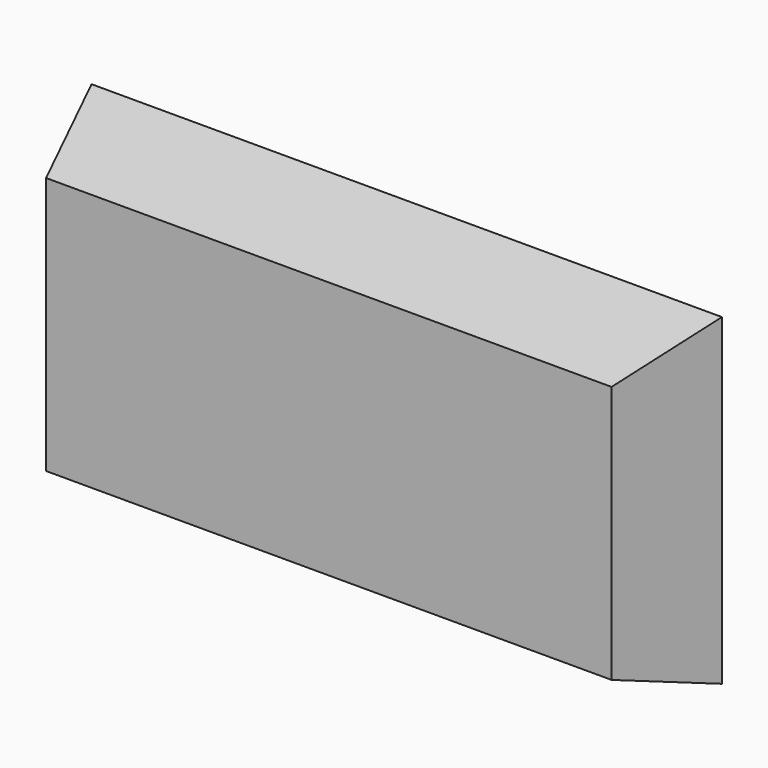
from build123d import *

# Parameters (mm, degrees)
F0_W     = 49.3294708431
F0_H     = 25.266315788
F1_DEPTH = 7.62
F2_SIZE2 = 7.61999
F2_SIZE  = 2.53999


# Not quite as in the source:
# - a fillet or chamfer is up to 0.001 mm smaller than in the source, because OpenCascade refuses the exact size


with BuildPart() as f1:
    # F0 (on Front) → F1 (new body)
    with BuildSketch(Plane.XZ):
        Rectangle(F0_W, F0_H)
    extrude(amount=F1_DEPTH)

    # F2 (size 2.54 and 7.62 in the source; OpenCascade refuses exactly that, so slightly less here)
    f2_edges = [f1.edges().sort_by_distance(p)[0] for p in [
        (0, -7.62, 12.633158),
        (24.664735, -7.62, 0),
        (-24.664735, -7.62, 0),
        (0, -7.62, -12.633158),
    ]]
    f2_side = f1.faces().sort_by_distance((0, -7.62, 0))[0]
    chamfer(f2_edges, length=F2_SIZE, length2=F2_SIZE2, reference=f2_side)


solid = f1.part
